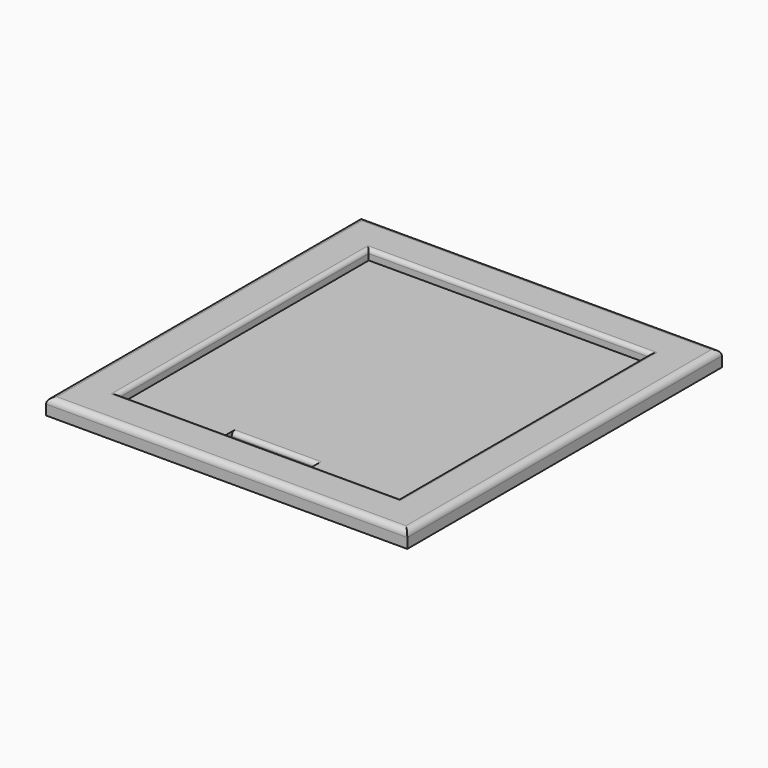
from build123d import *

# Parameters (mm, degrees)
F1_DEPTH = 1.5
F0_W     = 90
F0_H     = 98
F2_DEPTH = 4
F3_R     = 1
F4_R     = 1.5
F5_DEPTH = 3
F6_R     = 2


with BuildPart() as f1:
    # F0 (on Top) → F1 (new body)
    with BuildSketch(Plane.XY):
        Polygon((43.3765034378, 40.0858414471), (-26.6234965622, 40.0858414471), (-26.6234965622, -37.9141585529), (-2.3734965622, -37.9141585529), (-2.3734965622, -32.9141585529), (19.1265034378, -32.9141585529), (19.1265034378, -37.9141585529), (43.3765034378, -37.9141585529), align=None)
    extrude(amount=F1_DEPTH)

    # F0 (on Top) → F2 (join)
    with BuildSketch(Plane.XY):
        with Locations((8.3765034378, 1.0858414471)):
            Rectangle(F0_W, F0_H)
        with BuildLine():
            ThreePointArc((-31.6234965622, 42.5858414471), (-33.3912635152, 46.8536084001), (-29.1234965622, 45.0858414471))
            Line((-29.1234965622, 45.0858414471), (45.8765034378, 45.0858414471))
            ThreePointArc((45.8765034378, 45.0858414471), (48.3765034378, 47.5858414471), (50.8765034378, 45.0858414471))
            ThreePointArc((50.8765034378, 45.0858414471), (50.1442703907, 43.3180744941), (48.3765034378, 42.5858414471))
            Line((48.3765034378, 42.5858414471), (48.3765034378, -40.4141585529))
            ThreePointArc((48.3765034378, -40.4141585529), (50.1442703907, -41.1463915999), (50.8765034378, -42.9141585529))
            ThreePointArc((50.8765034378, -42.9141585529), (48.3765034378, -45.4141585529), (45.8765034378, -42.9141585529))
            Line((45.8765034378, -42.9141585529), (-29.1234965622, -42.9141585529))
            ThreePointArc((-29.1234965622, -42.9141585529), (-33.3912635152, -44.6819255059), (-31.6234965622, -40.4141585529))
            Line((-31.6234965622, -40.4141585529), (-31.6234965622, 42.5858414471))
        make_face(mode=Mode.SUBTRACT)
        with BuildLine():
            Line((-31.6234965622, -42.9141585529), (-31.6234965622, -40.4141585529))
            ThreePointArc((-31.6234965622, -40.4141585529), (-33.3912635152, -44.6819255059), (-29.1234965622, -42.9141585529))
            Line((-29.1234965622, -42.9141585529), (-31.6234965622, -42.9141585529))
        make_face()
        with BuildLine():
            Line((45.8765034378, 45.0858414471), (-29.1234965622, 45.0858414471))
            ThreePointArc((-29.1234965622, 45.0858414471), (-29.8557296093, 43.3180744941), (-31.6234965622, 42.5858414471))
            Line((-31.6234965622, 42.5858414471), (-31.6234965622, -40.4141585529))
            ThreePointArc((-31.6234965622, -40.4141585529), (-29.8557296093, -41.1463915999), (-29.1234965622, -42.9141585529))
            Line((-29.1234965622, -42.9141585529), (45.8765034378, -42.9141585529))
            ThreePointArc((45.8765034378, -42.9141585529), (46.6087364848, -41.1463915999), (48.3765034378, -40.4141585529))
            Line((48.3765034378, -40.4141585529), (48.3765034378, 42.5858414471))
            ThreePointArc((48.3765034378, 42.5858414471), (46.6087364848, 43.3180744941), (45.8765034378, 45.0858414471))
        make_face()
        Polygon((-26.6234965622, -37.9141585529), (-26.6234965622, 40.0858414471), (43.3765034378, 40.0858414471), (43.3765034378, -37.9141585529), (19.1265034378, -37.9141585529), (-2.3734965622, -37.9141585529), align=None, mode=Mode.SUBTRACT)
        with BuildLine():
            ThreePointArc((-29.1234965622, -42.9141585529), (-29.8557296093, -41.1463915999), (-31.6234965622, -40.4141585529))
            Line((-31.6234965622, -40.4141585529), (-31.6234965622, -42.9141585529))
            Line((-31.6234965622, -42.9141585529), (-29.1234965622, -42.9141585529))
        make_face()
        with BuildLine():
            ThreePointArc((50.8765034378, -42.9141585529), (50.1442703907, -41.1463915999), (48.3765034378, -40.4141585529))
            Line((48.3765034378, -40.4141585529), (48.3765034378, -42.9141585529))
            Line((48.3765034378, -42.9141585529), (45.8765034378, -42.9141585529))
            ThreePointArc((45.8765034378, -42.9141585529), (48.3765034378, -45.4141585529), (50.8765034378, -42.9141585529))
        make_face()
        with BuildLine():
            Line((48.3765034378, -42.9141585529), (48.3765034378, -40.4141585529))
            ThreePointArc((48.3765034378, -40.4141585529), (46.6087364848, -41.1463915999), (45.8765034378, -42.9141585529))
            Line((45.8765034378, -42.9141585529), (48.3765034378, -42.9141585529))
        make_face()
        with BuildLine():
            Line((48.3765034378, 45.0858414471), (45.8765034378, 45.0858414471))
            ThreePointArc((45.8765034378, 45.0858414471), (46.6087364848, 43.3180744941), (48.3765034378, 42.5858414471))
            Line((48.3765034378, 42.5858414471), (48.3765034378, 45.0858414471))
        make_face()
        with BuildLine():
            ThreePointArc((50.8765034378, 45.0858414471), (48.3765034378, 47.5858414471), (45.8765034378, 45.0858414471))
            Line((45.8765034378, 45.0858414471), (48.3765034378, 45.0858414471))
            Line((48.3765034378, 45.0858414471), (48.3765034378, 42.5858414471))
            ThreePointArc((48.3765034378, 42.5858414471), (50.1442703907, 43.3180744941), (50.8765034378, 45.0858414471))
        make_face()
        with BuildLine():
            Line((-31.6234965622, 42.5858414471), (-31.6234965622, 45.0858414471))
            Line((-31.6234965622, 45.0858414471), (-29.1234965622, 45.0858414471))
            ThreePointArc((-29.1234965622, 45.0858414471), (-33.3912635152, 46.8536084001), (-31.6234965622, 42.5858414471))
        make_face()
        with BuildLine():
            Line((-29.1234965622, 45.0858414471), (-31.6234965622, 45.0858414471))
            Line((-31.6234965622, 45.0858414471), (-31.6234965622, 42.5858414471))
            ThreePointArc((-31.6234965622, 42.5858414471), (-29.8557296093, 43.3180744941), (-29.1234965622, 45.0858414471))
        make_face()
    extrude(amount=F2_DEPTH)

    # F3
    f3_edges = [f1.edges().sort_by_distance(p)[0] for p in [
        (8.376503, -32.914159, 1.5),
        (-26.623497, 1.085841, 4),
        (8.376503, -37.914159, 4),
        (43.376503, 1.085841, 4),
        (8.376503, 40.085841, 4),
    ]]
    fillet(f3_edges, radius=F3_R)

    # F4
    f4_edges = [f1.edges().sort_by_distance(p)[0] for p in [
        (-36.623497, 1.085841, 4),
        (8.376503, 50.085841, 4),
        (53.376503, 1.085841, 4),
        (8.376503, -47.914159, 4),
    ]]
    fillet(f4_edges, radius=F4_R)

    # F0 (on Top) → F5 (cut)
    with BuildSketch(Plane.XY):
        with BuildLine():
            Line((48.3765034378, 45.0858414471), (45.8765034378, 45.0858414471))
            ThreePointArc((45.8765034378, 45.0858414471), (46.6087364848, 43.3180744941), (48.3765034378, 42.5858414471))
            Line((48.3765034378, 42.5858414471), (48.3765034378, 45.0858414471))
        make_face()
        with BuildLine():
            ThreePointArc((50.8765034378, 45.0858414471), (48.3765034378, 47.5858414471), (45.8765034378, 45.0858414471))
            Line((45.8765034378, 45.0858414471), (48.3765034378, 45.0858414471))
            Line((48.3765034378, 45.0858414471), (48.3765034378, 42.5858414471))
            ThreePointArc((48.3765034378, 42.5858414471), (50.1442703907, 43.3180744941), (50.8765034378, 45.0858414471))
        make_face()
        with BuildLine():
            Line((-31.6234965622, 42.5858414471), (-31.6234965622, 45.0858414471))
            Line((-31.6234965622, 45.0858414471), (-29.1234965622, 45.0858414471))
            ThreePointArc((-29.1234965622, 45.0858414471), (-33.3912635152, 46.8536084001), (-31.6234965622, 42.5858414471))
        make_face()
        with BuildLine():
            Line((-29.1234965622, 45.0858414471), (-31.6234965622, 45.0858414471))
            Line((-31.6234965622, 45.0858414471), (-31.6234965622, 42.5858414471))
            ThreePointArc((-31.6234965622, 42.5858414471), (-29.8557296093, 43.3180744941), (-29.1234965622, 45.0858414471))
        make_face()
        with BuildLine():
            Line((48.3765034378, -42.9141585529), (48.3765034378, -40.4141585529))
            ThreePointArc((48.3765034378, -40.4141585529), (46.6087364848, -41.1463915999), (45.8765034378, -42.9141585529))
            Line((45.8765034378, -42.9141585529), (48.3765034378, -42.9141585529))
        make_face()
        with BuildLine():
            ThreePointArc((50.8765034378, -42.9141585529), (50.1442703907, -41.1463915999), (48.3765034378, -40.4141585529))
            Line((48.3765034378, -40.4141585529), (48.3765034378, -42.9141585529))
            Line((48.3765034378, -42.9141585529), (45.8765034378, -42.9141585529))
            ThreePointArc((45.8765034378, -42.9141585529), (48.3765034378, -45.4141585529), (50.8765034378, -42.9141585529))
        make_face()
        with BuildLine():
            Line((-31.6234965622, -42.9141585529), (-31.6234965622, -40.4141585529))
            ThreePointArc((-31.6234965622, -40.4141585529), (-33.3912635152, -44.6819255059), (-29.1234965622, -42.9141585529))
            Line((-29.1234965622, -42.9141585529), (-31.6234965622, -42.9141585529))
        make_face()
        with BuildLine():
            ThreePointArc((-29.1234965622, -42.9141585529), (-29.8557296093, -41.1463915999), (-31.6234965622, -40.4141585529))
            Line((-31.6234965622, -40.4141585529), (-31.6234965622, -42.9141585529))
            Line((-31.6234965622, -42.9141585529), (-29.1234965622, -42.9141585529))
        make_face()
    extrude(amount=F5_DEPTH, mode=Mode.SUBTRACT)

    # F6
    f6_edges = [f1.edges().sort_by_distance(p)[0] for p in [
        (50.876503, -42.914159, 3),
        (48.376503, 47.585841, 3),
        (-31.623497, 47.585841, 3),
        (-34.123497, -42.914159, 3),
    ]]
    fillet(f6_edges, radius=F6_R)


solid = f1.part
